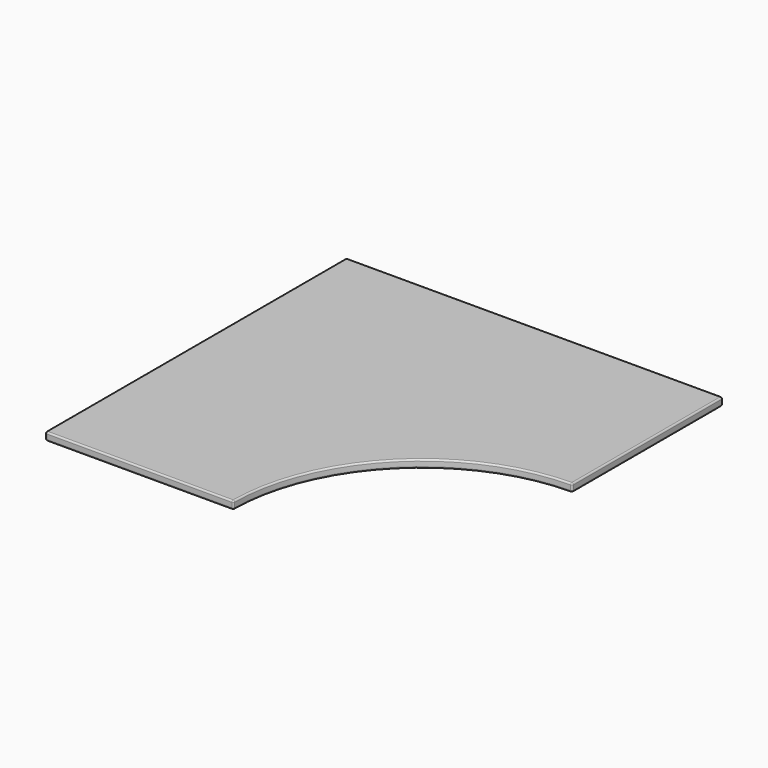
from build123d import *

# Parameters (mm, degrees)
F1_DEPTH = 25.4
F2_R     = 5.08
F3_R     = 5.08
F4_R     = 5.08
F5_R     = 5.08
F6_R     = 5.08
F9_R     = 5.08
F10_R    = 5.08


# Not quite as in the source:
# - the program builds the solid bodies; features that only make, move or delete a surface that nothing else refers to are left out


with BuildPart() as f1:
    # F0 (on Top) → F1 (new body)
    with BuildSketch(Plane.XY):
        with BuildLine():
            Line((596.8167068857, 124.9892751187), (596.8167068857, 724.9880751187))
            Line((596.8167068857, 724.9880751187), (-603.1832931143, 724.9880751187))
            Line((-603.1832931143, 724.9880751187), (-603.1832931143, -475.0095248813))
            Line((-603.1832931143, -475.0095248813), (-3.1820931143, -475.0095248813))
            ThreePointArc((-3.1820931143, -475.0095248813), (172.5534867019, -50.7463046975), (596.8167068857, 124.9892751187))
        make_face()
    extrude(amount=F1_DEPTH)

    # F2
    f2_edges = [f1.edges().sort_by_distance(p)[0] for p in [
        (-603.183293, -475.009525, 12.7),
    ]]
    fillet(f2_edges, radius=F2_R)

    # F3
    f3_edges = [f1.edges().sort_by_distance(p)[0] for p in [
        (-3.182093, -475.009525, 12.7),
    ]]
    fillet(f3_edges, radius=F3_R)

    # F4
    f4_edges = [f1.edges().sort_by_distance(p)[0] for p in [
        (596.816707, 124.989275, 12.7),
    ]]
    fillet(f4_edges, radius=F4_R)

    # F5
    f5_edges = [f1.edges().sort_by_distance(p)[0] for p in [
        (596.816707, 724.988075, 12.7),
    ]]
    fillet(f5_edges, radius=F5_R)

    # F6
    f6_edges = [f1.edges().sort_by_distance(p)[0] for p in [
        (-603.183293, 724.988075, 12.7),
    ]]
    fillet(f6_edges, radius=F6_R)

    # F9
    f9_edges = [f1.edges().sort_by_distance(p)[0] for p in [
        (-303.172031, -475.009525, 0),
    ]]
    fillet(f9_edges, radius=F9_R)

    # F10
    f10_edges = [f1.edges().sort_by_distance(p)[0] for p in [
        (-303.172031, -475.009525, 25.4),
    ]]
    fillet(f10_edges, radius=F10_R)


solid = f1.part
